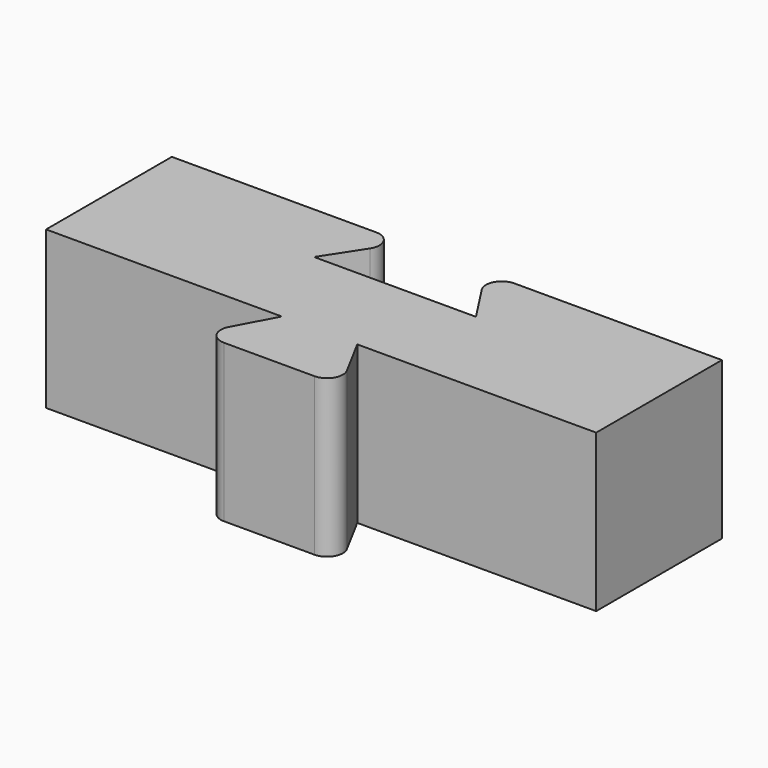
from build123d import *

# Parameters (mm, degrees)
F1_DEPTH = 10
F2_R     = 1


# Not quite as in the source:
# - a feature names something its author has since deleted; it is built from what else it names


with BuildPart() as f1:
    # F0 (on Top) → F1 (new body)
    with BuildSketch(Plane.XY):
        Polygon((2.3, -5), (17.5, -5), (17.5, 5), (2.45, 5), (5.05, 1), (-5.25, 1), (-2.65, 5), (-17.5, 5), (-17.5, -5), (-2.5, -5), align=None)
        Polygon((4.45, -9), (2.3, -5), (-2.5, -5), (-4.65, -9), align=None)
    extrude(amount=F1_DEPTH)

    # F2
    f2_edges = [f1.edges().sort_by_distance(p)[0] for p in [
        (-2.65, 5, 5),
        (2.45, 5, 5),
        (4.45, -9, 5),
        (-4.65, -9, 5),
    ]]
    fillet(f2_edges, radius=F2_R)


solid = f1.part
